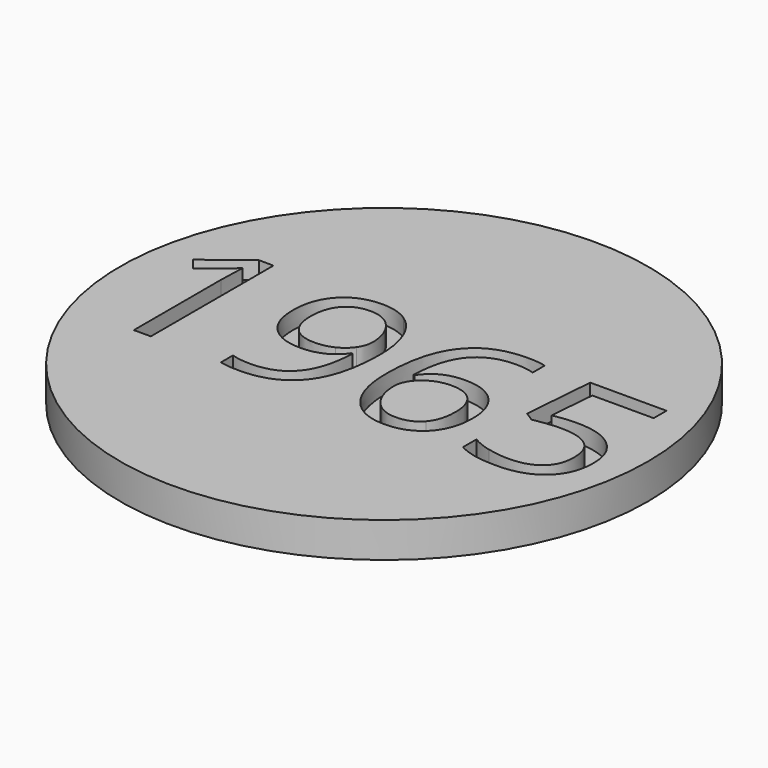
from build123d import *

# Parameters (mm, degrees)
F0_R         = 47.625
F1_DEPTH     = 6.35
F0_TEXT_SIZE = 38.7495743377
F2_DEPTH     = 3.175


# Not quite as in the source:
# - Text() gives the source's letters only with a copy of the font that has no kerning and outlines rounded to 1/6400 em; it was checked with that copy


with BuildPart() as f1:
    # F0 (on Top) → F1 (new body)
    with BuildSketch(Plane.XY):
        Circle(F0_R)
        with BuildLine():
            Line((-30.9239767078, 13.7084697814), (-30.9239767078, -13.9550935231))
            Line((-30.9239767078, -13.9550935231), (-33.9876149288, -13.9550935231))
            Line((-33.9876149288, -13.9550935231), (-33.9876149288, 5.7587524212))
            add(Edge.make_bspline(
                [(-33.9876149288, 5.7587524212), (-33.9876149288, 8.2229831642), (-33.8362494041, 10.4147559627)],
                knots=[0, 0, 0, 1, 1, 1], degree=2))
            add(Edge.make_bspline(
                [(-33.8362494041, 10.4147559627), (-34.2297997684, 10.0151509773), (-34.7232513791, 9.5822455765)],
                knots=[0, 0, 0, 1, 1, 1], degree=2))
            add(Edge.make_bspline(
                [(-34.7232513791, 9.5822455765), (-35.2167029899, 9.1493401757), (-39.2248620854, 5.891954083)],
                knots=[0, 0, 0, 1, 1, 1], degree=2))
            Line((-39.2248620854, 5.891954083), (-40.8898828577, 8.0473991555))
            Line((-40.8898828577, 8.0473991555), (-33.5698460805, 13.7084697814))
            Line((-33.5698460805, 13.7084697814), (-30.9239767078, 13.7084697814))
        make_face(mode=Mode.SUBTRACT)
        with BuildLine():
            add(Edge.make_bspline(
                [(-3.3542600286, 8.4379222094), (-2.2190185929, 5.6679331063), (-2.2190185929, 1.9019588504)],
                knots=[0, 0, 0, 1, 1, 1], degree=2))
            add(Edge.make_bspline(
                [(-2.2190185929, 1.9019588504), (-2.2190185929, -14.3365346455), (-14.7823571477, -14.3365346455)],
                knots=[0, 0, 0, 1, 1, 1], degree=2))
            add(Edge.make_bspline(
                [(-14.7823571477, -14.3365346455), (-16.9801845672, -14.3365346455), (-18.2637642171, -13.9550935231)],
                knots=[0, 0, 0, 1, 1, 1], degree=2))
            Line((-18.2637642171, -13.9550935231), (-18.2637642171, -11.2486779405))
            add(Edge.make_bspline(
                [(-18.2637642171, -11.2486779405), (-16.7501089696, -11.7391022407), (-14.8247394947, -11.7391022407)],
                knots=[0, 0, 0, 1, 1, 1], degree=2))
            add(Edge.make_bspline(
                [(-14.8247394947, -11.7391022407), (-10.283773752, -11.7391022407), (-7.9648539127, -8.9297581012)],
                knots=[0, 0, 0, 1, 1, 1], degree=2))
            add(Edge.make_bspline(
                [(-7.9648539127, -8.9297581012), (-5.6459340734, -6.1204139617), (-5.4400769597, -0.3140324321)],
                knots=[0, 0, 0, 1, 1, 1], degree=2))
            Line((-5.4400769597, -0.3140324321), (-5.6640979364, -0.3140324321))
            add(Edge.make_bspline(
                [(-5.6640979364, -0.3140324321), (-6.7054927467, -1.8821792685), (-8.4280324184, -2.7056077232)],
                knots=[0, 0, 0, 1, 1, 1], degree=2))
            add(Edge.make_bspline(
                [(-8.4280324184, -2.7056077232), (-10.1505720902, -3.5290361779), (-12.3060171627, -3.5290361779)],
                knots=[0, 0, 0, 1, 1, 1], degree=2))
            add(Edge.make_bspline(
                [(-12.3060171627, -3.5290361779), (-15.9751174828, -3.5290361779), (-18.1335898658, -1.3342360689)],
                knots=[0, 0, 0, 1, 1, 1], degree=2))
            add(Edge.make_bspline(
                [(-18.1335898658, -1.3342360689), (-20.2920622489, 0.86056404), (-20.2920622489, 4.7960676837)],
                knots=[0, 0, 0, 1, 1, 1], degree=2))
            add(Edge.make_bspline(
                [(-20.2920622489, 4.7960676837), (-20.2920622489, 9.1069578288), (-17.8792957842, 11.6044889873)],
                knots=[0, 0, 0, 1, 1, 1], degree=2))
            add(Edge.make_bspline(
                [(-17.8792957842, 11.6044889873), (-15.4665293196, 14.1020201457), (-11.531025676, 14.1020201457)],
                knots=[0, 0, 0, 1, 1, 1], degree=2))
            add(Edge.make_bspline(
                [(-11.531025676, 14.1020201457), (-8.7095722945, 14.1020201457), (-6.5995368794, 12.6549657291)],
                knots=[0, 0, 0, 1, 1, 1], degree=2))
            add(Edge.make_bspline(
                [(-6.5995368794, 12.6549657291), (-4.4895014643, 11.2079113124), (-3.3542600286, 8.4379222094)],
                knots=[0, 0, 0, 1, 1, 1], degree=2))
        make_face(mode=Mode.SUBTRACT)
        with BuildLine():
            add(Edge.make_bspline(
                [(4.5894027106, -11.1094216577), (2.0737076892, -7.8823086699), (2.0737076892, -2.1304187291)],
                knots=[0, 0, 0, 1, 1, 1], degree=2))
            add(Edge.make_bspline(
                [(2.0737076892, -2.1304187291), (2.0737076892, 6.0251557447), (5.2433017776, 10.0635879452)],
                knots=[0, 0, 0, 1, 1, 1], degree=2))
            add(Edge.make_bspline(
                [(5.2433017776, 10.0635879452), (8.412895866, 14.1020201457), (14.618882381, 14.1020201457)],
                knots=[0, 0, 0, 1, 1, 1], degree=2))
            add(Edge.make_bspline(
                [(14.618882381, 14.1020201457), (16.7561635905, 14.1020201457), (17.9852516516, 13.7447975073)],
                knots=[0, 0, 0, 1, 1, 1], degree=2))
            Line((17.9852516516, 13.7447975073), (17.9852516516, 11.0383819247))
            add(Edge.make_bspline(
                [(17.9852516516, 11.0383819247), (16.5260879929, 11.5106423619), (14.6552101069, 11.5106423619)],
                knots=[0, 0, 0, 1, 1, 1], degree=2))
            add(Edge.make_bspline(
                [(14.6552101069, 11.5106423619), (10.2050636791, 11.5106423619), (7.8588980454, 8.7406532589)],
                knots=[0, 0, 0, 1, 1, 1], degree=2))
            add(Edge.make_bspline(
                [(7.8588980454, 8.7406532589), (5.5127324116, 5.9706641558), (5.288711435, 0.0250263434)],
                knots=[0, 0, 0, 1, 1, 1], degree=2))
            Line((5.288711435, 0.0250263434), (5.5127324116, 0.0250263434))
            add(Edge.make_bspline(
                [(5.5127324116, 0.0250263434), (7.5955220323, 3.2824124362), (12.100160049, 3.2824124362)],
                knots=[0, 0, 0, 1, 1, 1], degree=2))
            add(Edge.make_bspline(
                [(12.100160049, 3.2824124362), (15.829806579, 3.2824124362), (17.9761697201, 1.0300934278)],
                knots=[0, 0, 0, 1, 1, 1], degree=2))
            add(Edge.make_bspline(
                [(17.9761697201, 1.0300934278), (20.1225328611, -1.2222255806), (20.1225328611, -5.0790191514)],
                knots=[0, 0, 0, 1, 1, 1], degree=2))
            add(Edge.make_bspline(
                [(20.1225328611, -5.0790191514), (20.1225328611, -9.3959639175), (17.7672852959, -11.8662492815)],
                knots=[0, 0, 0, 1, 1, 1], degree=2))
            add(Edge.make_bspline(
                [(17.7672852959, -11.8662492815), (15.4120377307, -14.3365346455), (11.3978240142, -14.3365346455)],
                knots=[0, 0, 0, 1, 1, 1], degree=2))
            add(Edge.make_bspline(
                [(11.3978240142, -14.3365346455), (7.1050977321, -14.3365346455), (4.5894027106, -11.1094216577)],
                knots=[0, 0, 0, 1, 1, 1], degree=2))
        make_face(mode=Mode.SUBTRACT)
        with BuildLine():
            add(Edge.make_bspline(
                [(28.2175611251, 2.5074209494), (30.3911700606, 2.9433536607), (32.5526697541, 2.9433536607)],
                knots=[0, 0, 0, 1, 1, 1], degree=2))
            add(Edge.make_bspline(
                [(32.5526697541, 2.9433536607), (36.9241061091, 2.9433536607), (39.4307191991, 0.7757993462)],
                knots=[0, 0, 0, 1, 1, 1], degree=2))
            add(Edge.make_bspline(
                [(39.4307191991, 0.7757993462), (41.937332289, -1.3917549683), (41.937332289, -5.1577292243)],
                knots=[0, 0, 0, 1, 1, 1], degree=2))
            add(Edge.make_bspline(
                [(41.937332289, -5.1577292243), (41.937332289, -9.4504555064), (39.2036709119, -11.8934950759)],
                knots=[0, 0, 0, 1, 1, 1], degree=2))
            add(Edge.make_bspline(
                [(39.2036709119, -11.8934950759), (36.4700095348, -14.3365346455), (31.6626404686, -14.3365346455)],
                knots=[0, 0, 0, 1, 1, 1], degree=2))
            add(Edge.make_bspline(
                [(31.6626404686, -14.3365346455), (26.9884730641, -14.3365346455), (24.530296942, -12.8410432609)],
                knots=[0, 0, 0, 1, 1, 1], degree=2))
            Line((24.530296942, -12.8410432609), (24.530296942, -9.8137327658))
            add(Edge.make_bspline(
                [(24.530296942, -9.8137327658), (25.8502043179, -10.6613797044), (27.8179561398, -11.1457493836)],
                knots=[0, 0, 0, 1, 1, 1], degree=2))
            add(Edge.make_bspline(
                [(27.8179561398, -11.1457493836), (29.7857079616, -11.6301190629), (31.6989681945, -11.6301190629)],
                knots=[0, 0, 0, 1, 1, 1], degree=2))
            add(Edge.make_bspline(
                [(31.6989681945, -11.6301190629), (35.0290097392, -11.6301190629), (36.8726418307, -10.0589449159)],
                knots=[0, 0, 0, 1, 1, 1], degree=2))
            add(Edge.make_bspline(
                [(36.8726418307, -10.0589449159), (38.7162739222, -8.4877707689), (38.7162739222, -5.5149518627)],
                knots=[0, 0, 0, 1, 1, 1], degree=2))
            add(Edge.make_bspline(
                [(38.7162739222, -5.5149518627), (38.7162739222, 0.273265804), (31.6263127426, 0.273265804)],
                knots=[0, 0, 0, 1, 1, 1], degree=2))
            add(Edge.make_bspline(
                [(31.6263127426, 0.273265804), (29.8280903085, 0.273265804), (26.8189436764, -0.2777047061)],
                knots=[0, 0, 0, 1, 1, 1], degree=2))
            Line((26.8189436764, -0.2777047061), (25.19025063, 0.7636901042))
            Line((25.19025063, 0.7636901042), (26.2316454403, 13.7084697814))
            Line((26.2316454403, 13.7084697814), (39.9877443302, 13.7084697814))
            Line((39.9877443302, 13.7084697814), (39.9877443302, 10.814360948))
            Line((39.9877443302, 10.814360948), (28.91989716, 10.814360948))
            Line((28.91989716, 10.814360948), (28.2175611251, 2.5074209494))
        make_face(mode=Mode.SUBTRACT)
    extrude(amount=F1_DEPTH)



with BuildPart() as f1b:
    # F0 (on Top) → F1, piece 2 (new body)
    with BuildSketch(Plane.XY):
        with BuildLine():
            add(Edge.make_bspline(
                [(-8.3432677246, 10.4541109991), (-9.7328032418, 11.4198230471), (-11.531025676, 11.4198230471)],
                knots=[0, 0, 0, 1, 1, 1], degree=2))
            add(Edge.make_bspline(
                [(-11.531025676, 11.4198230471), (-14.2374412586, 11.4198230471), (-15.7117414697, 9.6791195124)],
                knots=[0, 0, 0, 1, 1, 1], degree=2))
            add(Edge.make_bspline(
                [(-15.7117414697, 9.6791195124), (-17.1860416809, 7.9384159777), (-17.1860416809, 4.8323954097)],
                knots=[0, 0, 0, 1, 1, 1], degree=2))
            add(Edge.make_bspline(
                [(-17.1860416809, 4.8323954097), (-17.1860416809, 2.107815964), (-15.823751958, 0.548751059)],
                knots=[0, 0, 0, 1, 1, 1], degree=2))
            add(Edge.make_bspline(
                [(-15.823751958, 0.548751059), (-14.4614622352, -1.0103138459), (-11.6823912007, -1.0103138459)],
                knots=[0, 0, 0, 1, 1, 1], degree=2))
            add(Edge.make_bspline(
                [(-11.6823912007, -1.0103138459), (-9.9568242185, -1.0103138459), (-8.5097698018, -0.3110051216)],
                knots=[0, 0, 0, 1, 1, 1], degree=2))
            add(Edge.make_bspline(
                [(-8.5097698018, -0.3110051216), (-7.0627153851, 0.3883036028), (-6.230204999, 1.5992278009)],
                knots=[0, 0, 0, 1, 1, 1], degree=2))
            add(Edge.make_bspline(
                [(-6.230204999, 1.5992278009), (-5.3976946128, 2.8101519989), (-5.3976946128, 4.1361139958)],
                knots=[0, 0, 0, 1, 1, 1], degree=2))
            add(Edge.make_bspline(
                [(-5.3976946128, 4.1361139958), (-5.3976946128, 6.1220296806), (-6.1757134101, 7.8052143159)],
                knots=[0, 0, 0, 1, 1, 1], degree=2))
            add(Edge.make_bspline(
                [(-6.1757134101, 7.8052143159), (-6.9537322073, 9.4883989512), (-8.3432677246, 10.4541109991)],
                knots=[0, 0, 0, 1, 1, 1], degree=2))
        make_face()
    extrude(amount=F1_DEPTH)


with BuildPart() as f1c:
    # F0 (on Top) → F1, piece 3 (new body)
    with BuildSketch(Plane.XY):
        with BuildLine():
            add(Edge.make_bspline(
                [(8.1919021998, -10.6825708779), (9.5814377171, -11.6664467888), (11.3614962882, -11.6664467888)],
                knots=[0, 0, 0, 1, 1, 1], degree=2))
            add(Edge.make_bspline(
                [(11.3614962882, -11.6664467888), (14.0497480079, -11.6664467888), (15.5331301505, -9.9711529115)],
                knots=[0, 0, 0, 1, 1, 1], degree=2))
            add(Edge.make_bspline(
                [(15.5331301505, -9.9711529115), (17.0165122931, -8.2758590343), (17.0165122931, -5.0790191514)],
                knots=[0, 0, 0, 1, 1, 1], degree=2))
            add(Edge.make_bspline(
                [(17.0165122931, -5.0790191514), (17.0165122931, -2.3362758428), (15.6360587073, -0.7651016958)],
                knots=[0, 0, 0, 1, 1, 1], degree=2))
            add(Edge.make_bspline(
                [(15.6360587073, -0.7651016958), (14.2556051216, 0.8060724511), (11.512861813, 0.8060724511)],
                knots=[0, 0, 0, 1, 1, 1], degree=2))
            add(Edge.make_bspline(
                [(11.512861813, 0.8060724511), (9.8115133147, 0.8060724511), (8.3917046925, 0.1037364163)],
                knots=[0, 0, 0, 1, 1, 1], degree=2))
            add(Edge.make_bspline(
                [(8.3917046925, 0.1037364163), (6.9718960703, -0.5985996186), (6.1303037526, -1.8276876796)],
                knots=[0, 0, 0, 1, 1, 1], degree=2))
            add(Edge.make_bspline(
                [(6.1303037526, -1.8276876796), (5.288711435, -3.0567757407), (5.288711435, -4.3827377375)],
                knots=[0, 0, 0, 1, 1, 1], degree=2))
            add(Edge.make_bspline(
                [(5.288711435, -4.3827377375), (5.288711435, -6.3323256964), (6.0455390588, -8.0155103317)],
                knots=[0, 0, 0, 1, 1, 1], degree=2))
            add(Edge.make_bspline(
                [(6.0455390588, -8.0155103317), (6.8023666826, -9.698694967), (8.1919021998, -10.6825708779)],
                knots=[0, 0, 0, 1, 1, 1], degree=2))
        make_face()
    extrude(amount=F1_DEPTH)


with BuildPart() as f1_1:
    add(f1.part)

    add(f1b.part)  # F2 merges F1b

    add(f1c.part)  # F2 merges F1c
    # F0 (on Top) → F2 (join)
    with BuildSketch(Plane.XY):
        with Locations((-44.45, -13.9550935231)):
            Text('1965', F0_TEXT_SIZE, font='Open Sans', text_align=(TextAlign.LEFT, TextAlign.BOTTOM))
    extrude(amount=F2_DEPTH)


solid = f1_1.part
